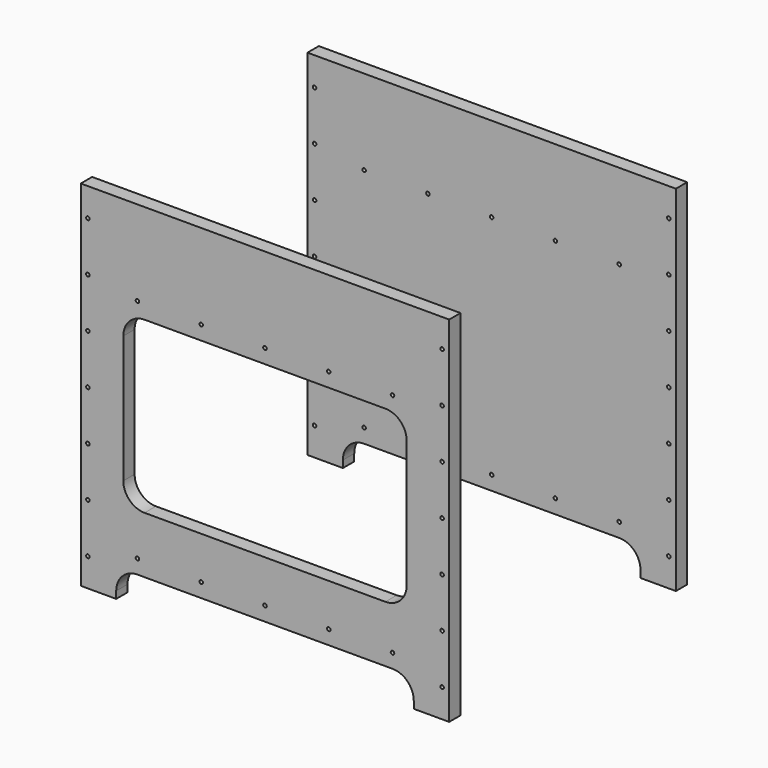
from build123d import *

# Parameters (mm, degrees)
F0_W     = 520
F0_H     = 500
F1_DEPTH = 20
F2_W     = 210
F2_H     = 40
F3_DEPTH = 20
F4_R     = 30
F6_W     = 200
F6_H     = 240
F7_DEPTH = 20
F8_R     = 30
F10_D    = 5
F10_2_D  = 5
F12_D    = 5
F12_2_D  = 5


# Not quite as in the source:
# - a feature names something its author has since deleted; it is built from what else it names


with BuildPart() as f1:
    # F0 (on Front) → F1 (new body)
    with BuildSketch(Plane.XZ):
        with Locations((23.5411918163, -8.8762454689)):
            Rectangle(F0_W, F0_H)
    extrude(amount=F1_DEPTH)

    # F2 (on face) → F3 (cut, through all)
    with BuildSketch(Plane.XZ.offset(20)):
        with Locations((-81.4588081837, -238.8762454689)):
            Rectangle(F2_W, F2_H)
        with Locations((128.5411918163, -238.8762454689)):
            Rectangle(F2_W, F2_H)
    extrude(amount=-F3_DEPTH, mode=Mode.SUBTRACT)

    # F4
    f4_edges = [f1.edges().sort_by_distance(p)[0] for p in [
        (-186.458808, -10, -218.876245),
        (233.541192, -10, -218.876245),
    ]]
    fillet(f4_edges, radius=F4_R)


with BuildPart() as f5_1:
    # F5: copy of F1
    add(f1.part.moved(Location((0, 400, 0))))

    # F10#2 (through all)
    with Locations(Plane.XZ.offset(20)):
        with Locations((-226.4588081837, 201.1237545311), (-226.4588081837, 131.1237545311), (-226.4588081837, 61.1237545311), (-226.4588081837, -8.8762454689), (-226.4588081837, -78.8762454689), (-226.4588081837, -148.8762454689), (273.5411918163, -218.8762454689), (273.5411918163, -148.8762454689), (273.5411918163, -78.8762454689), (273.5411918163, -8.8762454689), (273.5411918163, 61.1237545311), (273.5411918163, 131.1237545311), (273.5411918163, 201.1237545311), (-226.4588081837, -218.8762454689)):
            Hole(F10_2_D / 2)

    # F12#2 (through all)
    with Locations(Plane.XZ.offset(20)):
        with Locations((-156.4588081837, 121.1237545311), (-66.4588081837, 121.1237545311), (23.5411918163, 121.1237545311), (113.5411918163, 121.1237545311), (203.5411918163, 121.1237545311), (203.5411918163, -198.8762454689), (113.5411918163, -198.8762454689), (23.5411918163, -198.8762454689), (-66.4588081837, -198.8762454689), (-156.4588081837, -198.8762454689)):
            Hole(F12_2_D / 2)


with BuildPart() as f1_1:
    add(f1.part)

    # F6 (on face) → F7 (cut, through all)
    with BuildSketch(Plane.XZ.offset(20)):
        with Locations((-76.4588081837, -18.8762454689)):
            Rectangle(F6_W, F6_H)
        with Locations((123.5411918163, -18.8762454689)):
            Rectangle(F6_W, F6_H)
    extrude(amount=-F7_DEPTH, mode=Mode.SUBTRACT)

    # F8
    f8_edges = [f1_1.edges().sort_by_distance(p)[0] for p in [
        (-176.458808, -10, 101.123755),
        (-176.458808, -10, -138.876245),
        (223.541192, -10, 101.123755),
        (223.541192, -10, -138.876245),
    ]]
    fillet(f8_edges, radius=F8_R)

    # F10 (through all)
    with Locations(Plane.XZ.offset(20)):
        with Locations((-226.4588081837, 201.1237545311), (-226.4588081837, 131.1237545311), (-226.4588081837, 61.1237545311), (-226.4588081837, -8.8762454689), (-226.4588081837, -78.8762454689), (-226.4588081837, -148.8762454689), (273.5411918163, -218.8762454689), (273.5411918163, -148.8762454689), (273.5411918163, -78.8762454689), (273.5411918163, -8.8762454689), (273.5411918163, 61.1237545311), (273.5411918163, 131.1237545311), (273.5411918163, 201.1237545311), (-226.4588081837, -218.8762454689)):
            Hole(F10_D / 2)

    # F12 (through all)
    with Locations(Plane.XZ.offset(20)):
        with Locations((-156.4588081837, 121.1237545311), (-66.4588081837, 121.1237545311), (23.5411918163, 121.1237545311), (113.5411918163, 121.1237545311), (203.5411918163, 121.1237545311), (203.5411918163, -198.8762454689), (113.5411918163, -198.8762454689), (23.5411918163, -198.8762454689), (-66.4588081837, -198.8762454689), (-156.4588081837, -198.8762454689)):
            Hole(F12_D / 2)


solid = Compound([f5_1.part, f1_1.part])
